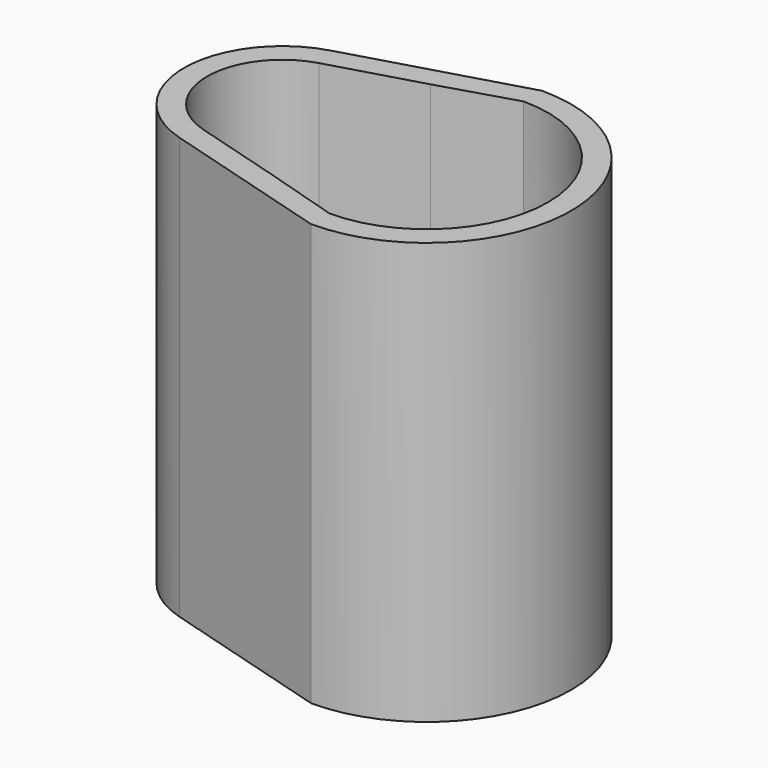
from build123d import *

# Parameters (mm, degrees)
F1_DEPTH  = 30
F3_DEPTH  = 27
F2_R      = 4
F5_DEPTH  = 6.5
F4_R      = 4.25
F4_R_2    = 4
F6_DEPTH  = 35.2
F7_DEPTH  = 10
F8_W      = 1
F8_H      = 16.5
F9_DEPTH  = 13.4
F11_DEPTH = 16
F12_DEPTH = 0.5
F13_R     = 1.25
F14_DEPTH = 25
F15_DEPTH = 2
F16_DEPTH = 18.5
F18_DEPTH = 15


with BuildPart() as f1:
    # F0 (on Top) → F1 (new body)
    with BuildSketch(Plane.XY):
        with BuildLine():
            ThreePointArc((-9.61, 7.9936162029), (-5.5424501439, 4.8828782496), (-4, 0))
            ThreePointArc((-4, 0), (-5.5424501439, -4.8828782496), (-9.61, -7.9936162029))
            ThreePointArc((-9.61, -7.9936162029), (-8.2636700449, -9.3787929602), (-6.72, -10.54))
            Line((-6.72, -10.54), (0, -12.5))
            ThreePointArc((0, -12.5), (8.8388347648, -8.8388347648), (12.5, 0))
            ThreePointArc((12.5, 0), (8.8388347648, 8.8388347648), (0, 12.5))
            Line((0, 12.5), (-6.72, 10.54))
            ThreePointArc((-6.72, 10.54), (-8.2636700449, 9.3787929602), (-9.61, 7.9936162029))
        make_face()
        with BuildLine():
            ThreePointArc((-4, 0), (0, 4), (4, 0))
            ThreePointArc((4, 0), (0, -4), (-4, 0))
        make_face(mode=Mode.SUBTRACT)
        with BuildLine():
            ThreePointArc((-9.61, -7.9936162029), (-5.5424501439, -4.8828782496), (-4, 0))
            ThreePointArc((-4, 0), (-5.5424501439, 4.8828782496), (-9.61, 7.9936162029))
            ThreePointArc((-9.61, 7.9936162029), (-12.5, 0), (-9.61, -7.9936162029))
        make_face()
        with BuildLine():
            ThreePointArc((-14.88, 8.16), (-12.231772686, 8.4957668346), (-9.61, 7.9936162029))
            ThreePointArc((-9.61, 7.9936162029), (-8.2636700449, 9.3787929602), (-6.72, 10.54))
            Line((-6.72, 10.54), (-14.88, 8.16))
        make_face()
        with BuildLine():
            ThreePointArc((-9.61, -7.9936162029), (-12.5, 0), (-9.61, 7.9936162029))
            ThreePointArc((-9.61, 7.9936162029), (-12.231772686, 8.4957668346), (-14.88, 8.16))
            ThreePointArc((-14.88, 8.16), (-21, 0), (-14.88, -8.16))
            ThreePointArc((-14.88, -8.16), (-12.231772686, -8.4957668346), (-9.61, -7.9936162029))
        make_face()
        with BuildLine():
            ThreePointArc((-6.72, -10.54), (-8.2636700449, -9.3787929602), (-9.61, -7.9936162029))
            ThreePointArc((-9.61, -7.9936162029), (-12.231772686, -8.4957668346), (-14.88, -8.16))
            Line((-14.88, -8.16), (-6.72, -10.54))
        make_face()
    extrude(amount=F1_DEPTH)

    # F2 (on face) → F3 (cut)
    with BuildSketch(Plane.XY.offset(30)):
        with BuildLine():
            Line((-14.32, -6.24), (-6.5, -8.5208333333))
            Line((-6.5, -8.5208333333), (-6.5, -6.5))
            Line((-6.5, -6.5), (-6.5, 6.5))
            Line((-6.5, 6.5), (-6.5, 8.5208333333))
            Line((-6.5, 8.5208333333), (-14.32, 6.24))
            ThreePointArc((-14.32, 6.24), (-19, 0), (-14.32, -6.24))
        make_face()
    extrude(amount=-F3_DEPTH, mode=Mode.SUBTRACT)

    # F2 (on face) → F5 (cut)
    with BuildSketch(Plane.XY.offset(30)):
        Polygon((-6.5, 6.5), (-6.5, -6.5), (6.5, -6.5), (10, 0), (6.5, 6.5), align=None)
        Circle(F2_R, mode=Mode.SUBTRACT)
    extrude(amount=-F5_DEPTH, mode=Mode.SUBTRACT)

    # F4 (on face) → F6 (cut)
    with BuildSketch(Plane.XY.offset(30)):
        Circle(F4_R)
        Circle(F4_R_2, mode=Mode.SUBTRACT)
    extrude(amount=-F6_DEPTH, mode=Mode.SUBTRACT)

    # F7 (add): a face of the model
    f7_faces = [f1.faces().sort_by_distance(p)[0] for p in [
        (-7.3229596651, 9.9287188517, 30),
    ]]
    extrude(f7_faces, amount=F7_DEPTH)

    # F8 (on face) → F9 (join)
    with BuildSketch(Plane.XZ.offset(-6.5)):
        with Locations((-6, 31.75)):
            Rectangle(F8_W, F8_H)
    extrude(amount=F9_DEPTH)

    # F10 (on face) → F11 (cut)
    with BuildSketch(Plane.XY.offset(40)):
        with BuildLine():
            Line((6.5, -6.5), (-5.5, -6.5))
            Line((-5.5, -6.5), (0, -12.5))
            ThreePointArc((0, -12.5), (12.5, 0), (0, 12.5))
            Line((0, 12.5), (-5.5, 6.5))
            Line((-5.5, 6.5), (6.5, 6.5))
            Line((6.5, 6.5), (10, 0))
            Line((10, 0), (6.5, -6.5))
        make_face()
    extrude(amount=-F11_DEPTH, mode=Mode.SUBTRACT)

    # F12 (cut): a face of the model
    f12_faces = [f1.faces().sort_by_distance(p)[0] for p in [
        (0.5, -6.808058436, 24),
    ]]
    extrude(f12_faces, amount=-F12_DEPTH, mode=Mode.SUBTRACT)

    # F13 (on face) → F14 (cut)
    with BuildSketch(Plane.YZ.offset(-5.5)):
        with Locations((0, 31.75)):
            Circle(F13_R)
    extrude(amount=-F14_DEPTH, mode=Mode.SUBTRACT)

    # F15 (cut): a face of the model
    f15_faces = [f1.faces().sort_by_distance(p)[0] for p in [
        (-2.5229134485, -9.2918373278, 23.5),
    ]]
    extrude(f15_faces, amount=-F15_DEPTH, mode=Mode.SUBTRACT)

    # F16 (cut): a face of the model
    f16_faces = [f1.faces().sort_by_distance(p)[0] for p in [
        (-2.9906782868, 9.7206217629, 40),
    ]]
    extrude(f16_faces, amount=-F16_DEPTH, mode=Mode.SUBTRACT)

    # F17 (on face) → F18 (join)
    with BuildSketch(Plane.XY.offset(21.5)):
        with BuildLine():
            ThreePointArc((-14.88, 8.16), (-21, 0), (-14.88, -8.16))
            Line((-14.88, -8.16), (0, -12.5))
            ThreePointArc((0, -12.5), (12.5, 0), (0, 12.5))
            Line((0, 12.5), (-14.88, 8.16))
        make_face()
        with BuildLine():
            ThreePointArc((0, 10.5), (10.5, 0), (0, -10.5))
            Line((0, -10.5), (-6.5, -8.5208333333))
            Line((-6.5, -8.5208333333), (-14.32, -6.24))
            ThreePointArc((-14.32, -6.24), (-19, 0), (-14.32, 6.24))
            Line((-14.32, 6.24), (-6.5, 8.5208333333))
            Line((-6.5, 8.5208333333), (0, 10.5))
        make_face(mode=Mode.SUBTRACT)
    extrude(amount=F18_DEPTH)


solid = f1.part
